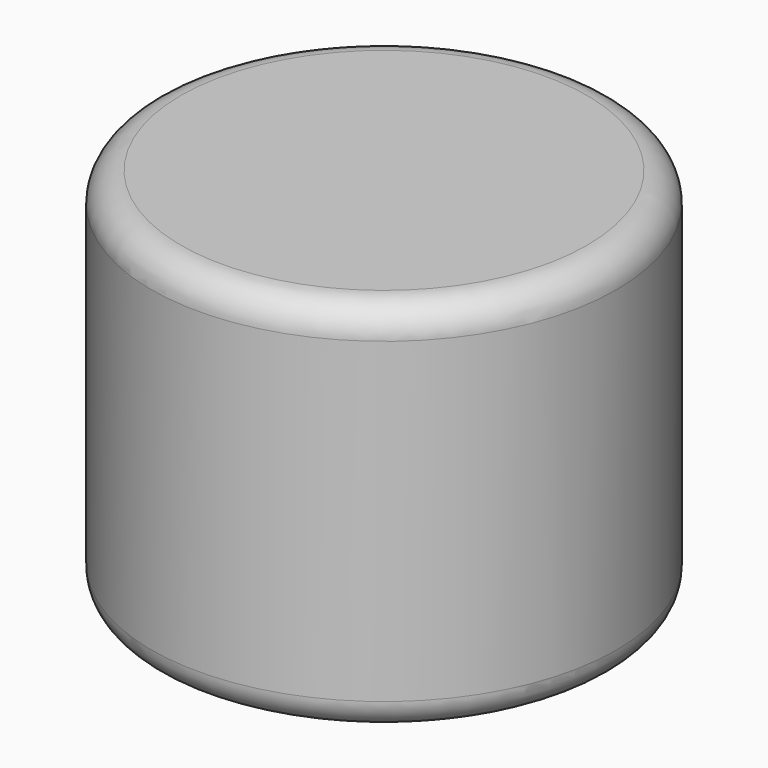
from build123d import *

# Parameters (mm, degrees)
F0_R     = 40.0419350947
F0_R_2   = 20.0959383488
F1_DEPTH = 64.77
F6_R     = 5.08


# Not quite as in the source:
# - the program builds the solid bodies; features that only make, move or delete a surface that nothing else refers to are left out


with BuildPart() as f1:
    # F0 (on Top) → F1 (new body)
    with BuildSketch(Plane.XY):
        Circle(F0_R)
        Circle(F0_R_2, mode=Mode.SUBTRACT)
        Circle(F0_R_2)
    extrude(amount=-F1_DEPTH)

    # F6
    f6_edges = [f1.edges().sort_by_distance(p)[0] for p in [
        (40.041935, 0, -32.385),
        (-40.041935, 0, 0),
        (-40.041935, 0, -64.77),
    ]]
    fillet(f6_edges, radius=F6_R)


solid = f1.part
